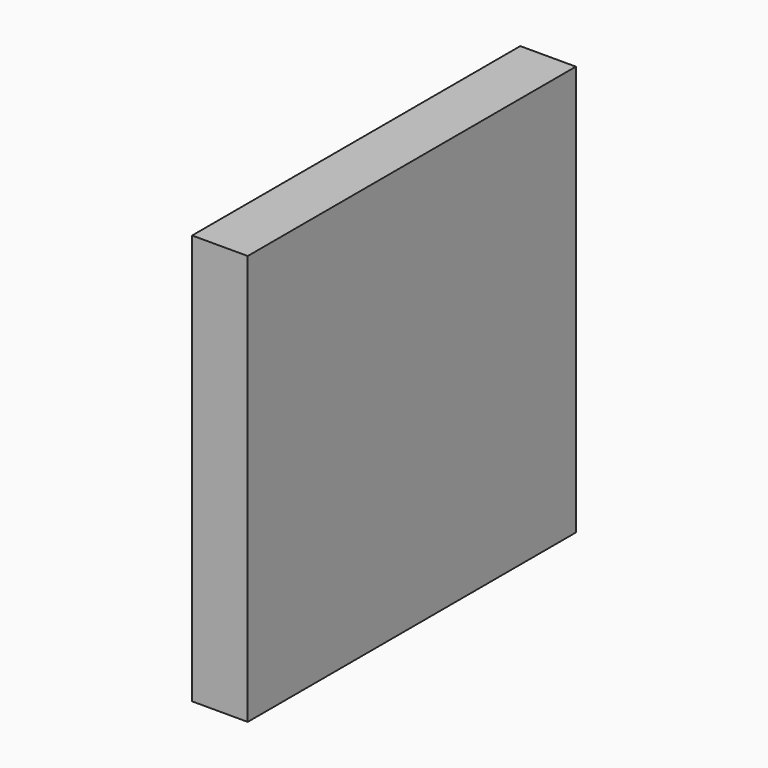
from build123d import *

# Parameters (mm, degrees)
F2_W     = 184.3985915184
F2_H     = 184.3985915184
F9_DEPTH = 25


# Not quite as in the source:
# - the program builds the solid bodies; features that only make, move or delete a surface that nothing else refers to are left out


with BuildPart() as f9:
    # F2 (on offset) → F9 (new body)
    with BuildSketch(Plane.YZ.offset(100)):
        Rectangle(F2_W, F2_H)
    extrude(amount=F9_DEPTH)


solid = f9.part
